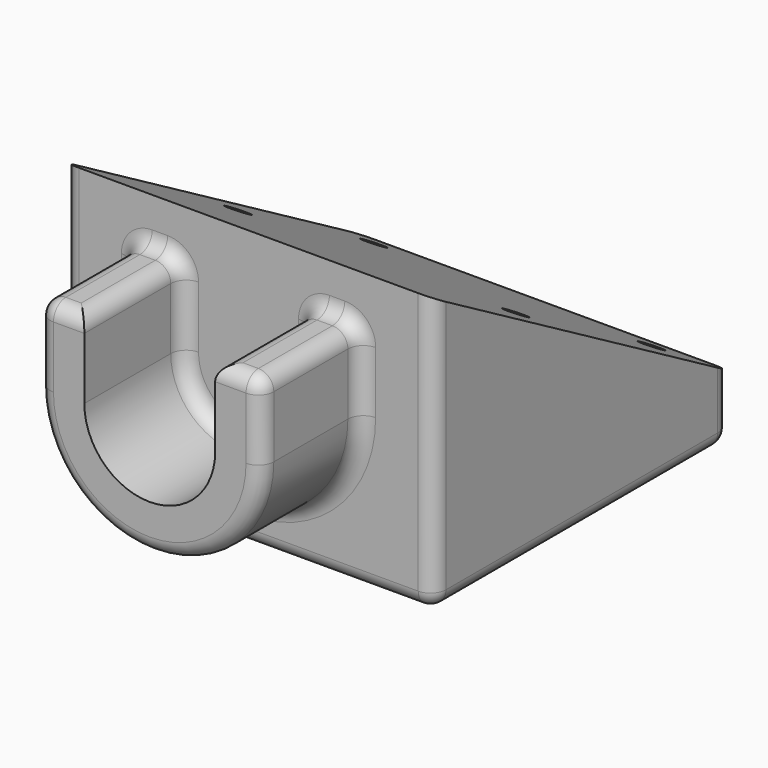
from build123d import *

# Parameters (mm, degrees)
F1_DEPTH = 38.1
F3_D     = 4.699
F5_R     = 3.175
F7_D     = 8.255
F7_DEPTH = 38.1
F7_TIP   = 2.480052205
F9_DEPTH = 25.4
F10_R    = 3.175


with BuildPart() as f1:
    # F0 (on Right) → F1 (new body, symmetric)
    with BuildSketch(Plane.YZ):
        Polygon((-38.1, 31.75), (-38.1, -25.4), (38.1, -25.4), (38.1, -12.2440905122), align=None)
    extrude(amount=F1_DEPTH, both=True)

    # F3 (through all)
    with Locations(Plane(origin=(0, 4.2231532851, 7.3147160579), x_dir=(1, 0, 0), z_dir=(0, 0.5, 0.8660254038))):
        with Locations((28.575, -10.7705678842), (-28.575, -10.7705678842), (-28.575, 29.5926131403), (28.575, 29.5926131403)):
            Hole(F3_D / 2)

    # F5
    f5_edges = [f1.edges().sort_by_distance(p)[0] for p in [
        (-38.1, -38.1, 3.175),
        (0, -38.1, -25.4),
        (38.1, -38.1, 3.175),
        (-38.1, 0, -25.4),
        (38.1, 0, -25.4),
        (0, 38.1, -25.4),
        (38.1, 38.1, -18.822045),
        (-38.1, 38.1, -18.822045),
    ]]
    fillet(f5_edges, radius=F5_R)

    # F7
    with Locations(Plane(origin=(0, -21.1768467149, -36.6793744543), x_dir=(1, 0, 0), z_dir=(0, -0.5, -0.8660254038))):
        with Locations((-28.575, 10.7705678842), (28.575, 10.7705678842), (28.575, -29.5926131403), (-28.575, -29.5926131403)):
            Hole(F7_D / 2, depth=F7_DEPTH)
            with Locations((0, 0, -(F7_DEPTH + F7_TIP / 2))):  # 118° drill point
                Cone(0, F7_D / 2, F7_TIP, mode=Mode.SUBTRACT)

    # F8 (on face) → F9 (join)
    with BuildSketch(Plane.XZ.offset(38.1)):
        with BuildLine():
            ThreePointArc((13.462, 6.35), (0, -7.112), (-13.462, 6.35))
            Line((-13.462, 6.35), (-13.462, 22.225))
            Line((-13.462, 22.225), (-22.987, 22.225))
            Line((-22.987, 22.225), (-22.987, 6.35))
            ThreePointArc((-22.987, 6.35), (0, -16.637), (22.987, 6.35))
            Line((22.987, 6.35), (22.987, 22.225))
            Line((22.987, 22.225), (13.462, 22.225))
            Line((13.462, 22.225), (13.462, 6.35))
        make_face()
    extrude(amount=F9_DEPTH)

    # F10
    f10_edges = [f1.edges().sort_by_distance(p)[0] for p in [
        (0, -38.1, -16.637),
        (0, -63.5, -16.637),
        (-18.2245, -38.1, 22.225),
        (18.2245, -38.1, 22.225),
        (-22.987, -50.8, 22.225),
        (-13.462, -50.8, 22.225),
        (13.462, -50.8, 22.225),
        (-18.2245, -63.5, 22.225),
        (18.2245, -63.5, 22.225),
        (22.987, -50.8, 22.225),
        (0, -38.1, -7.112),
        (-13.462, -38.1, 14.2875),
        (-22.987, -38.1, 14.2875),
        (22.987, -38.1, 14.2875),
        (13.462, -38.1, 14.2875),
        (-22.987, -63.5, 14.2875),
        (22.987, -63.5, 14.2875),
    ]]
    fillet(f10_edges, radius=F10_R)


solid = f1.part
